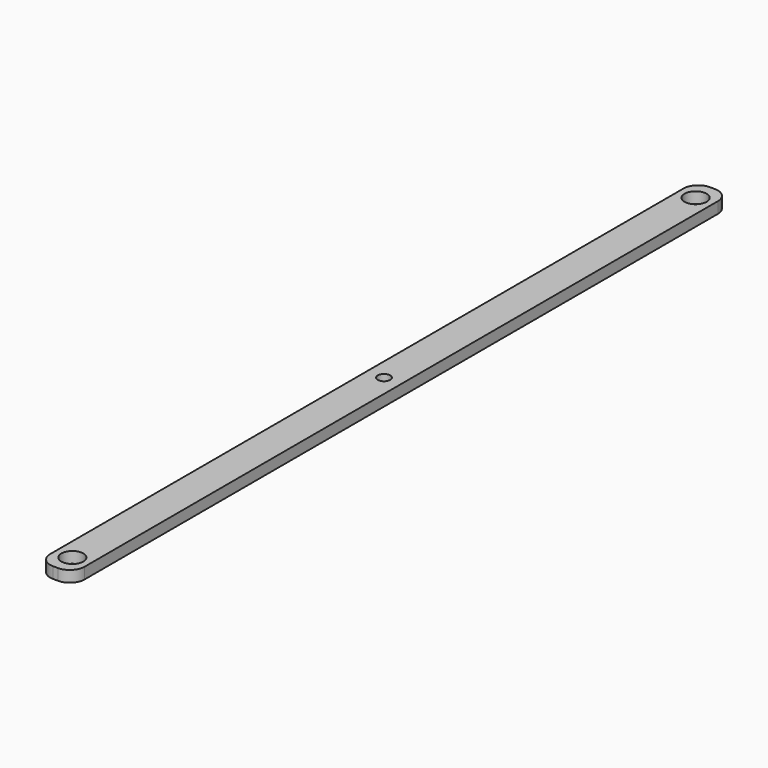
from build123d import *

# Parameters (mm, degrees)
F0_W          = 5.9313117526
F0_H          = 1.9345532637
F1_DEPTH      = 70.8533
F1_DEPTH_BACK = 70.8533
F2_R          = 2.54
F3_R          = 1.9022356475
F4_DEPTH      = 2.3622
F5_R          = 1.0755010134
F6_DEPTH      = 2.01676


# Not quite as in the source:
# - a pattern or mirror of a feature is missing from the dataset's text; its kind, count and spacing are read off the source's solid


with BuildPart() as f1:
    # F0 (on Front) → F1 (new body, two sides)
    with BuildSketch(Plane.XZ) as f1_sk:
        Rectangle(F0_W, F0_H)
    extrude(amount=F1_DEPTH)
    extrude(f1_sk.sketch, amount=-F1_DEPTH_BACK)

    # F2
    f2_edges = [f1.edges().sort_by_distance(p)[0] for p in [
        (2.965656, -70.8533, 0),
        (-2.965656, -70.8533, 0),
        (2.965656, 70.8533, 0),
        (-2.965656, 70.8533, 0),
    ]]
    fillet(f2_edges, radius=F2_R)

    # F3 (on face) → F4 (cut)
    with BuildSketch(Plane.XY.offset(0.9672766319)):
        with Locations((0, 67.2314763069)):
            Circle(F3_R)
    f4 = extrude(amount=-F4_DEPTH, mode=Mode.SUBTRACT)

    # F4_copies: F4 across plane
    add(f4.mirror(Plane(origin=(0, 0, 0), x_dir=(0, 0, -1), z_dir=(0, -1, 0))), mode=Mode.SUBTRACT)

    # F5 (on face) → F6 (cut)
    with BuildSketch(Plane.XY.offset(0.9672766319)):
        Circle(F5_R)
    extrude(amount=-F6_DEPTH, mode=Mode.SUBTRACT)


solid = f1.part
